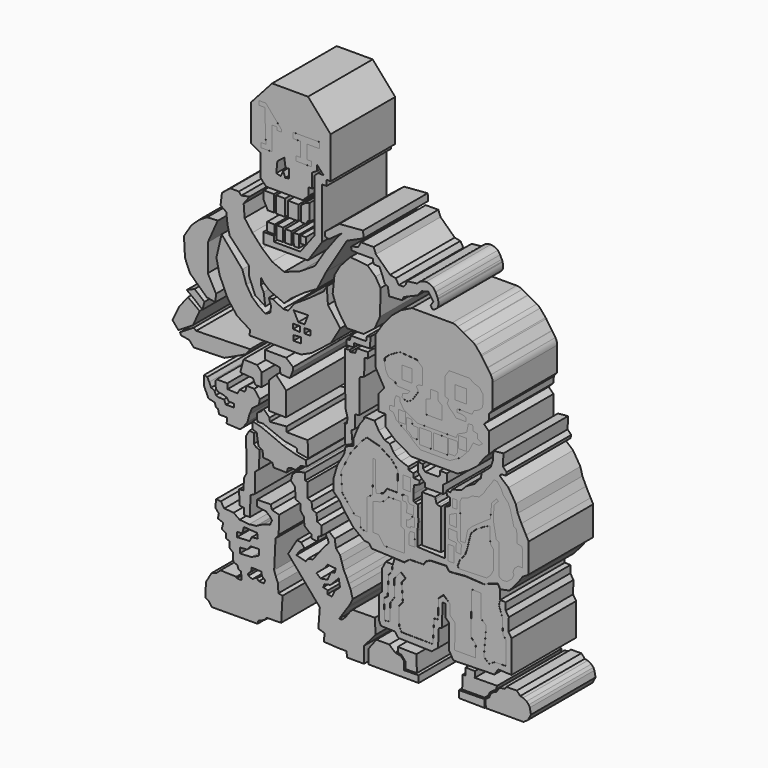
from build123d import *

# Parameters (mm, degrees)
F1_DEPTH       = 12.7
F1_DEPTH_BACK  = 12.7
F0_W           = 2.3451782763
F0_H           = 2.7289353311
F3_DEPTH       = 12.7
F3_DEPTH_BACK  = 12.7
F2_W           = 3.1842617318
F2_H           = 4.0236283094
F2_W_2         = 3.6299433559
F2_H_2         = 4.2267246172
F2_W_3         = 1.8677245826
F2_H_3         = 4.6415366232
F2_W_4         = 1.5032105148
F2_H_4         = 2.5777257979
F2_W_5         = 3.182772547
F2_H_5         = 4.0222080424
F2_W_6         = 3.6285351962
F2_H_6         = 4.2254780419
F2_W_7         = 2.2105854005
F2_H_7         = 3.4294971265
F2_W_8         = 1.8693469465
F2_H_8         = 4.6432167292
F2_W_9         = 1.5042312443
F2_H_9         = 2.5786831975
F2_W_10        = 3.7808120251
F2_H_10        = 4.7481860965
F2_W_11        = 4.3708886951
F2_H_11        = 4.6935402788
F2_W_12        = 2.4654623121
F2_H_12        = 3.6471767817
F2_W_13        = 2.2135460749
F2_H_13        = 3.4322766587
F2_W_14        = 3.7859473377
F2_H_14        = 4.7525740229
F2_W_15        = 4.3766628951
F2_H_15        = 4.6988725662
F2_W_16        = 2.4702642113
F2_H_16        = 3.651695326
F4_T1_DEPTH    = 33.1807281465
F4_T3_DEPTH    = 32.7857254502
F4_T5_DEPTH    = 26.7239636698
F4_T7_DEPTH    = 28.894725654
F4_T9_DEPTH    = 32.1217717721
F4_T11_DEPTH   = 35.0005666731
F4_2_T1_DEPTH  = 25.4
F4_2_T3_DEPTH  = 30.6299842336
F4_2_T5_DEPTH  = 25.6431743127
F4_2_T7_DEPTH  = 26.2196872845
F4_2_T9_DEPTH  = 28.8182396822
F4_2_T11_DEPTH = 30.1563360546


# Not quite as in the source:
# - a fillet or chamfer that OpenCascade refuses, or shapes differently, is made with other operations: its cross-section is extruded or revolved along the edge and cut away or added
# - a feature names something its author has since deleted; it is built from what else it names


with BuildPart() as f1:
    # F0 (on Front) → F1 (new body, two sides)
    with BuildSketch(Plane.XZ) as f1_sk:
        Polygon((-9.5938611776, 66.9106543064), (-16.6862662882, 74.9939456582), (-27.994306758, 74.9939456582), (-34.6385799348, 67.5830319524), (-34.6385799348, 56.2110990286), (-31.6603220999, 54.5591711998), (-31.6603220999, 47.6847961545), (-29.7909770161, 45.815449208), (-18.3336883783, 45.815449208), (-16.5246427059, 47.5641936064), (-16.5246427059, 49.9762557447), (-15.3789138421, 49.9762557447), (-15.3789138421, 54.4385686517), (-13.9103056863, 55.3104877472), (-13.9103056863, 57.1270510554), (-11.8339713663, 54.8590533435), (-13.5205361214, 54.8850011104), (-14.5949935541, 53.9049506187), (-14.5949935541, 37.3129360378), (-17.3938885863, 33.6037576199), (-19.1130582243, 31.3254632056), (-27.4183992296, 31.3254632056), (-27.4183992296, 32.9865328968), (-30.7405348867, 32.9865328968), (-30.7405348867, 29.6643972397), (-16.7492311448, 29.6643972397), (-12.3410113156, 36.1170060933), (-12.3410113156, 52.1527044475), (-10.8716050163, 52.1527044475), (-10.8716050163, 53.877659142), (-9.5938611776, 53.877659142), align=None)
        Polygon((-26.3316370547, 54.0427602828), (-24.165680632, 55.7010732591), (-23.7595625222, 52.9597811401), (-22.728053189, 53.1125976231), (-22.728053189, 50.3538660705), (-23.861091584, 50.2184927464), (-24.5041102171, 51.8768019974), (-25.3163445741, 50.184648484), (-26.6700685024, 50.5569241941), align=None, mode=Mode.SUBTRACT)
        Polygon((-31.4840041101, 57.4934072793), (-29.9422182143, 57.4934072793), (-30.3007718176, 67.6046609879), (-32.0935472846, 67.6046609879), (-32.0935472846, 68.8936337829), (-29.9574602395, 68.8936337829), (-24.9686259777, 63.0946457386), (-24.9686259777, 62.4657310545), (-26.4403745532, 62.4657310545), (-26.5174116939, 63.4554550052), (-28.077730909, 63.4554550052), (-28.077730909, 56.0591891408), (-31.4840041101, 56.0591891408), align=None, mode=Mode.SUBTRACT)
        Polygon((-21.3707555085, 61.8773698807), (-21.3707555085, 63.4141266346), (-21.3707555085, 63.6133402586), (-13.1177809089, 63.6133402586), (-13.1177809089, 61.763536185), (-16.9881414622, 61.763536185), (-16.9881414622, 57.4662983418), (-15.6221324578, 57.4662983418), (-15.6221324578, 55.9295378625), (-20.4316228628, 55.9295378625), (-20.4316228628, 57.4093796313), (-19.0371554345, 57.4093796313), (-19.0371554345, 61.8773698807), align=None, mode=Mode.SUBTRACT)
    extrude(amount=F1_DEPTH)
    extrude(f1_sk.sketch, amount=-F1_DEPTH_BACK)


with BuildPart() as f1b:
    # F0 (on Front) → F1, piece 2 (new body, two sides)
    with BuildSketch(Plane.XZ) as f1_2_sk:
        Polygon((-30.6372623891, 44.5467084646), (-30.6372623891, 44.2908704281), (-30.6372623891, 41.903052479), (-29.358074069, 39.4299551845), (-27.3966528475, 39.4299551845), (-27.3966528475, 44.5467084646), align=None)
    extrude(amount=F1_DEPTH)
    extrude(f1_2_sk.sketch, amount=-F1_DEPTH_BACK)


with BuildPart() as f1c:
    # F0 (on Front) → F1, piece 3 (new body, two sides)
    with BuildSketch(Plane.XZ) as f1_3_sk:
        Polygon((-23.9142030478, 44.4402880967), (-26.7252419144, 44.472232461), (-26.7252419144, 39.3612533808), (-23.9142030478, 39.3612533808), align=None)
    extrude(amount=F1_DEPTH)
    extrude(f1_3_sk.sketch, amount=-F1_DEPTH_BACK)


with BuildPart() as f1d:
    # F0 (on Front) → F1, piece 4 (new body, two sides)
    with BuildSketch(Plane.XZ) as f1_4_sk:
        Polygon((-19.6976456791, 44.1527962685), (-22.9558944702, 44.1847406328), (-22.9558944702, 39.5529158413), (-19.6976456791, 39.5529158413), align=None)
    extrude(amount=F1_DEPTH)
    extrude(f1_4_sk.sketch, amount=-F1_DEPTH_BACK)


with BuildPart() as f1e:
    # F0 (on Front) → F1, piece 5 (new body, two sides)
    with BuildSketch(Plane.XZ) as f1_5_sk:
        Polygon((-17.4935366958, 45.2708229423), (-18.8671126962, 44.2805700004), (-18.8671126962, 39.5529158413), (-17.1741005033, 39.5529158413), (-16.8227199465, 40.5431687832), (-16.1519050598, 40.5431687832), (-16.1519050598, 45.7819215953), align=None)
    extrude(amount=F1_DEPTH)
    extrude(f1_5_sk.sketch, amount=-F1_DEPTH_BACK)


with BuildPart() as f1f:
    # F0 (on Front) → F1, piece 6 (new body, two sides)
    with BuildSketch(Plane.XZ) as f1_6_sk:
        Polygon((-19.0333388746, 33.6037576199), (-17.3938885863, 33.6037576199), (-17.3938885863, 35.8636565506), (-19.0333388746, 35.8636565506), (-19.0333388746, 35.5651788414), align=None)
    extrude(amount=F1_DEPTH)
    extrude(f1_6_sk.sketch, amount=-F1_DEPTH_BACK)


with BuildPart() as f1g:
    # F0 (on Front) → F1, piece 7 (new body, two sides)
    with BuildSketch(Plane.XZ) as f1_7_sk:
        Polygon((-21.2505981326, 35.8636565506), (-21.1653206497, 32.1540087461), (-19.5450149477, 32.1540087461), (-19.5450149477, 35.8636565506), align=None)
    extrude(amount=F1_DEPTH)
    extrude(f1_7_sk.sketch, amount=-F1_DEPTH_BACK)


with BuildPart() as f1h:
    # F0 (on Front) → F1, piece 8 (new body, two sides)
    with BuildSketch(Plane.XZ) as f1_8_sk:
        Polygon((-23.8516163081, 36.0342152417), (-23.8942559808, 32.1966484189), (-21.8475535512, 32.1966484189), (-21.8475535512, 36.0342152417), align=None)
    extrude(amount=F1_DEPTH)
    extrude(f1_8_sk.sketch, amount=-F1_DEPTH_BACK)


with BuildPart() as f1i:
    # F0 (on Front) → F1, piece 9 (new body, two sides)
    with BuildSketch(Plane.XZ) as f1_9_sk:
        Polygon((-26.5379119664, 36.2047739327), (-26.623191312, 32.1966484189), (-24.5338492095, 32.1966484189), (-24.5338492095, 36.2047739327), align=None)
    extrude(amount=F1_DEPTH)
    extrude(f1_9_sk.sketch, amount=-F1_DEPTH_BACK)


with BuildPart() as f1j:
    # F0 (on Front) → F1, piece 10 (new body, two sides)
    with BuildSketch(Plane.XZ) as f1_10_sk:
        with Locations((-28.3500943333, 34.8403062671)):
            Rectangle(F0_W, F0_H)
    extrude(amount=F1_DEPTH)
    extrude(f1_10_sk.sketch, amount=-F1_DEPTH_BACK)


with BuildPart() as f1k:
    # F0 (on Front) → F1, piece 11 (new body, two sides)
    with BuildSketch(Plane.XZ) as f1_11_sk:
        Polygon((-36.9369212724, 38.8479313689), (-35.0333526731, 41.3705967367), (-37.6954227686, 40.775667876), (-38.418225944, 41.6791699827), (-41.128732264, 41.6791699827), (-43.7488853931, 39.6011136472), (-44.2006364465, 35.9871052206), (-42.3936359584, 34.7222052515), (-42.0322343707, 31.4695984125), (-41.3094311953, 28.488041833), (-35.2559685707, 22.1635270864), (-35.2559685707, 19.3626713008), (-33.3586148918, 14.6644618362), (-30.1060080528, 12.5864073634), (-30.6481085718, 16.3811147213), (-31.5516106784, 18.097769469), (-31.42894949, 20.0820728757), (-30.6238532066, 18.9463123679), (-28.6898408085, 17.3346363008), (-24.1771470755, 15.4006257653), (-21.9745226204, 17.4420811236), (-17.7304428071, 20.4505436122), (-13.8624189422, 22.7068904787), (-10.961400345, 28.4014809877), (-4.491341766, 39.0913411975), (0.7715018001, 41.4606525215), (0.5989942583, 43.5738749802), (-6.8465704098, 42.9660752416), (-11.3291051239, 39.3952429295), (-11.3291051239, 38.0276888609), (-10.1135037839, 37.7237871289), (-6.0868188739, 40.610846132), (-7.7582728118, 38.7114658952), (-11.4810559899, 33.6971059442), (-14.5200621337, 28.8346949965), (-19.1545449197, 25.8716642857), (-24.1689067334, 24.0482613444), (-27.9676634818, 25.6437398493), (-31.0826450586, 28.3028688282), (-34.1976247728, 31.6457748413), (-36.6288311779, 34.9127091467), align=None)
    extrude(amount=F1_DEPTH)
    extrude(f1_11_sk.sketch, amount=-F1_DEPTH_BACK)


with BuildPart() as f1l:
    # F0 (on Front) → F1, piece 12 (new body, two sides)
    with BuildSketch(Plane.XZ) as f1_12_sk:
        Polygon((-0.9377481183, 38.5080315173), (-3.0890780035, 37.9343405366), (-3.1607891433, 37.7909205854), (-2.9456561897, 36.9303897023), (-1.2245918624, 36.7869660258), (3.723466536, 36.7869660258), (3.8668890484, 35.3527478874), (5.8030853979, 35.2093242109), (6.663617678, 33.2014150918), (7.3807276785, 31.1935078353), (8.3846813068, 30.6198205799), (8.8149476796, 28.0382242054), (12.8307631239, 28.2533578575), (13.4044513106, 29.3290223926), (15.0538031012, 30.0461333245), (17.7788212895, 31.1935078353), (18.9979076385, 32.7711515129), (21.1492385715, 33.3448387682), (22.7268803865, 31.0500860214), (21.8663476408, 29.8309996724), (22.4400348961, 28.7553351372), (23.6591231078, 29.0421787649), (24.5913658291, 30.7632423937), (24.0176785737, 32.6277278364), (23.0854358524, 34.5639251173), (21.7229258269, 35.7830114663), (18.4959303588, 35.7830114663), (17.6354013383, 34.4205051661), (14.4084058702, 34.0619497001), (13.978138566, 32.9145714641), (13.4044513106, 32.1974642575), (11.8268085644, 32.1257524192), (10.894565843, 33.7033942342), (9.1017913073, 34.0619497001), (4.6557090245, 38.2928960025), (3.938599024, 40.0856733322), (0, 40.0856733322), align=None)
    extrude(amount=F1_DEPTH)
    extrude(f1_12_sk.sketch, amount=-F1_DEPTH_BACK)

    # F4: fillet of radius 3.5186609131 on 6 edges, made by hand

    # F4_s2 → F4_t1 (cut)
    with BuildSketch(Plane.XZ.offset(-16.5903640732)):
        with BuildLine():
            ThreePointArc((24.400289, 30.4104851414), (23.576390538, 29.3978829612), (22.4400348961, 28.7553351372))
            Line((22.4400348961, 28.7553351372), (22.4627084207, 28.6887145614))
            ThreePointArc((22.4627084207, 28.6887145614), (23.065697202, 28.830254444), (23.6752413078, 28.9736762579))
            Line((23.6752413078, 28.9736762579), (23.7210017144, 29.0086611891))
            Line((23.7210017144, 29.0086611891), (24.4621676066, 30.3769675656))
            Line((24.4621676066, 30.3769675656), (24.400289, 30.4104851414))
        make_face()
    extrude(amount=F4_T1_DEPTH, mode=Mode.SUBTRACT)

    # F4_s4 → F4_t3 (cut)
    with BuildSketch(Plane.XZ.offset(-16.3928627251)):
        with BuildLine():
            ThreePointArc((24.1569587579, 32.1750667856), (24.2953412231, 30.792633601), (23.8878265601, 29.4644005581))
            Line((23.8878265601, 29.4644005581), (23.9497051667, 29.4308829823))
            Line((23.9497051667, 29.4308829823), (24.6673152211, 30.7557016546))
            Line((24.6673152211, 30.7557016546), (24.2242200085, 32.1957625344))
            Line((24.2242200085, 32.1957625344), (24.1569587579, 32.1750667856))
        make_face()
    extrude(amount=F4_T3_DEPTH, mode=Mode.SUBTRACT)

    # F4_s6 → F4_t5 (cut)
    with BuildSketch(Plane.XZ.offset(-13.3619818349)):
        with BuildLine():
            ThreePointArc((23.9028073914, 32.8663065517), (24.0084156505, 32.6240965562), (24.0955502986, 32.3746444777))
            Line((24.0955502986, 32.3746444777), (24.1628115492, 32.3953402265))
            Line((24.1628115492, 32.3953402265), (24.0833823898, 32.6534852523))
            Line((24.0833823898, 32.6534852523), (23.9662137839, 32.896835542))
            Line((23.9662137839, 32.896835542), (23.9028073914, 32.8663065517))
        make_face()
    extrude(amount=F4_T5_DEPTH, mode=Mode.SUBTRACT)

    # F4_s8 → F4_t7 (cut)
    with BuildSketch(Plane.XZ.offset(-14.447362827)):
        with BuildLine():
            ThreePointArc((22.5645527671, 35.0299778045), (23.030491922, 34.5226046703), (23.3886490575, 33.9341743347))
            Line((23.3886490575, 33.9341743347), (23.45205545, 33.9647033249))
            Line((23.45205545, 33.9647033249), (23.1427779808, 34.6070491231))
            Line((23.1427779808, 34.6070491231), (22.6114772337, 35.0824228641))
            Line((22.6114772337, 35.0824228641), (22.5645527671, 35.0299778045))
        make_face()
    extrude(amount=F4_T7_DEPTH, mode=Mode.SUBTRACT)

    # F4_s10 → F4_t9 (cut)
    with BuildSketch(Plane.XZ.offset(-16.060885886)):
        with BuildLine():
            ThreePointArc((20.3785714725, 35.7830114663), (21.6343890455, 35.5512787308), (22.724794805, 34.886603534))
            Line((22.724794805, 34.886603534), (22.7717192716, 34.9390485936))
            Line((22.7717192716, 34.9390485936), (21.749812914, 35.8533846845))
            Line((21.749812914, 35.8533846845), (20.3785714725, 35.8533846845))
            Line((20.3785714725, 35.8533846845), (20.3785714725, 35.7830114663))
        make_face()
    extrude(amount=F4_T9_DEPTH, mode=Mode.SUBTRACT)

    # F4_s12 → F4_t11 (cut)
    with BuildSketch(Plane.XZ.offset(-17.5002833365)):
        with BuildLine():
            ThreePointArc((17.6354013383, 34.4205051661), (18.8677869862, 35.4240777234), (20.4160436934, 35.7830114663))
            Line((20.4160436934, 35.7830114663), (20.4160436934, 35.8533846845))
            Line((20.4160436934, 35.8533846845), (18.4959303588, 35.8533846845))
            Line((18.4959303588, 35.8533846845), (18.4364305585, 35.8205902318))
            ThreePointArc((18.4364305585, 35.8205902318), (18.0061660483, 35.1393370817), (17.5797884912, 34.4636282583))
            Line((17.5797884912, 34.4636282583), (17.6354013383, 34.4205051661))
        make_face()
    extrude(amount=F4_T11_DEPTH, mode=Mode.SUBTRACT)


with BuildPart() as f1m:
    # F0 (on Front) → F1, piece 13 (new body, two sides)
    with BuildSketch(Plane.XZ) as f1_13_sk:
        Polygon((2.0290226676, 34.3684926629), (-3.3819169391, 34.9032784963), (-5.0103398971, 33.2014150918), (-6.7701800726, 31.1195589602), (-8.394648321, 28.276739642), (-8.936136961, 22.9972191155), (-7.8531587496, 20.0190264732), (-6.0933185741, 17.1085204929), (-4.4688507915, 14.8748783395), (0.8106696187, 15.0102507323), (4.1949781589, 17.5823252648), (5.9548197314, 21.508121863), (6.0901925899, 29.4274035841), (4.5334086753, 32.0671647787), align=None)
    extrude(amount=F1_DEPTH)
    extrude(f1_13_sk.sketch, amount=-F1_DEPTH_BACK)


with BuildPart() as f1n:
    # F0 (on Front) → F1, piece 14 (new body, two sides)
    with BuildSketch(Plane.XZ) as f1_14_sk:
        Polygon((-37.35839203, 20.4856079072), (-43.8636057079, 28.0750244856), (-45.4980805516, 21.0728552192), (-44.4747321308, 16.553055495), (-41.9163554907, 10.8393486589), (-39.0168614686, 7.087062113), (-34.9234566092, 4.5286854729), (-35.0940153003, 2.908379538), (-18.8909620047, 2.908379538), (-15.6503524631, 4.3581272475), (-9.5305331051, 9.1014830396), (-6.5489741974, 14.1610940918), (-10.4340352118, 19.4014050066), (-10.7954340056, 24.3706665933), (-11.7892883718, 22.6540118456), (-16.6681967676, 19.1303547472), (-20.8243075758, 16.4198484272), (-22.9927096516, 13.7093439698), (-24.5286636055, 13.7093439698), (-27.7812685817, 15.335646458), (-29.0461741388, 15.335646458), (-28.323372826, 13.2575919852), (-28.5944230855, 11.2698879093), (-30.1303770393, 10.5470865965), (-32.2987772524, 11.9926892221), (-34.2864841223, 13.7996925041), (-36.0934883356, 16.6908986866), align=None)
        Polygon((-21.2671738118, 5.9554395266), (-21.2671738118, 7.5206770562), (-18.9672354609, 7.7123385854), (-18.9672354609, 5.9554395266), align=None, mode=Mode.SUBTRACT)
        Polygon((-21.3949494064, 9.1498009861), (-21.3949494064, 10.6511516497), (-19.1588960588, 10.6511516497), (-19.1588960588, 8.9900828898), align=None, mode=Mode.SUBTRACT)
        Polygon((-19.7437535971, 11.6068609059), (-20.9376644343, 13.9094004408), (-21.1935024709, 14.4210755825), (-16.6737027466, 14.506354928), (-17.7823323756, 11.6068609059), align=None, mode=Mode.SUBTRACT)
        Polygon((-17.8172644228, 9.0539706871), (-17.8172644228, 10.5872638524), (-15.9006472677, 10.6511516497), (-15.9006472677, 9.0539706871), align=None, mode=Mode.SUBTRACT)
    extrude(amount=F1_DEPTH)
    extrude(f1_14_sk.sketch, amount=-F1_DEPTH_BACK)


with BuildPart() as f1o:
    # F0 (on Front) → F1, piece 15 (new body, two sides)
    with BuildSketch(Plane.XZ) as f1_15_sk:
        Polygon((-48.2119210064, 24.4022365659), (-45.1531931758, 31.3246250153), (-44.9922047555, 31.4856097102), (-48.4028458595, 31.2973856926), (-50.9676299989, 29.741641134), (-53.3509030938, 27.4967011064), (-55.6977577507, 23.7582940608), (-55.3757883608, 17.8018212318), (-53.8464225829, 14.0991490334), (-50.7876947522, 11.2014058977), (-48.5338903964, 9.1085908934), (-45.7971356809, 8.6256340146), (-45.636150986, 11.0404202715), (-48.2119210064, 15.8699918538), align=None)
    extrude(amount=F1_DEPTH)
    extrude(f1_15_sk.sketch, amount=-F1_DEPTH_BACK)


with BuildPart() as f1p:
    # F0 (on Front) → F1, piece 16 (new body, two sides)
    with BuildSketch(Plane.XZ) as f1_16_sk:
        Polygon((-52.33906582, 10.1660164073), (-54.8434145749, 9.0845925733), (-52.5667332113, 7.4339979328), (-49.8916320503, 5.2142329514), (-49.2655448616, 7.6047494076), align=None)
    extrude(amount=F1_DEPTH)
    extrude(f1_16_sk.sketch, amount=-F1_DEPTH_BACK)


with BuildPart() as f1q:
    # F0 (on Front) → F1, piece 17 (new body, two sides)
    with BuildSketch(Plane.XZ) as f1_17_sk:
        Polygon((-50.790656358, 4.5965607278), (-54.4437915087, 7.2289654054), (-57.129919529, 3.7907224614), (-59.3325421214, -0.6682488602), (-57.4522539973, -2.8708733153), (-52.8321154416, 0), align=None)
    extrude(amount=F1_DEPTH)
    extrude(f1_17_sk.sketch, amount=-F1_DEPTH_BACK)


with BuildPart() as f1r:
    # F0 (on Front) → F1, piece 18 (new body, two sides)
    with BuildSketch(Plane.XZ) as f1_18_sk:
        Polygon((-52.617225796, -0.6145262741), (-56.9150298834, -3.3006537706), (-56.6464141011, -4.0527693927), (-54.0677346289, -4.4825496152), (-52.617225796, -6.094226148), (-43.0546104908, -5.8793355711), (-39.5626462996, -4.267659504), (-36.2318493426, -2.655983204), (-34.8887853324, -0.8294165018), (-51.8651083112, -1.2591967825), align=None)
    extrude(amount=F1_DEPTH)
    extrude(f1_18_sk.sketch, amount=-F1_DEPTH_BACK)


with BuildPart() as f1s:
    # F0 (on Front) → F1, piece 19 (new body, two sides)
    with BuildSketch(Plane.XZ) as f1_19_sk:
        Polygon((-23.6031040549, 0.4885619273), (-30.1950573921, 0.5392691819), (-30.1950573921, -2.1482193843), (-25.5299843848, -2.8074146248), (-25.3778602928, -4.5821708627), (-22.4875435233, -4.7850008123), (-21.524105221, -2.7567071375), (-21.3719829917, -1.3876094017), align=None)
    extrude(amount=F1_DEPTH)
    extrude(f1_19_sk.sketch, amount=-F1_DEPTH_BACK)


with BuildPart() as f1t:
    # F0 (on Front) → F1, piece 20 (new body, two sides)
    with BuildSketch(Plane.XZ) as f1_20_sk:
        Polygon((-36.8002168834, -4.3107029051), (-36.9612015784, -4.3107029051), (-38.0076095462, -8.2548540086), (-33.9829660952, -8.5768252611), (-33.2585312426, -10.1866824552), (-31.3267037272, -10.1866824552), (-31.2462095171, -6.0815461911), (-32.695081085, -4.4716885313), align=None)
    extrude(amount=F1_DEPTH)
    extrude(f1_20_sk.sketch, amount=-F1_DEPTH_BACK)


with BuildPart() as f1u:
    # F0 (on Front) → F1, piece 21 (new body, two sides)
    with BuildSketch(Plane.XZ) as f1_21_sk:
        Polygon((-28.9138779044, -7.434383966), (-29.0096011013, -7.434383966), (-29.0096011013, -15.9537047148), (-23.6491281539, -16.049426049), (-23.5534086823, -8.5830567405), (-26.7122555524, -5.2327625453), align=None)
    extrude(amount=F1_DEPTH)
    extrude(f1_21_sk.sketch, amount=-F1_DEPTH_BACK)


with BuildPart() as f1v:
    # F0 (on Front) → F1, piece 22 (new body, two sides)
    with BuildSketch(Plane.XZ) as f1_22_sk:
        Polygon((-5.1528443582, -11.6437776014), (-4.9752146006, -17.6448337734), (-2.6907407378, -16.5448998462), (-3.0455661472, -12.9111642018), (-1.8998369342, -12.1272439137), (-1.929987804, -8.1473439932), (-0.5732035497, -7.9362886027), (-0.42929349, 2.6036400814), (0.9762255359, 3.2425122336), (0.9992049308, 8.3681419492), (2.2052354179, 8.7299505249), (2.0846324041, 10.4183927178), (-1.2922529131, 10.3580914438), (-1.8349663587, 8.9108552784), (-3.40280612, 8.6394986138), (-3.5535597708, 9.21236258), (-5.0912485458, 8.9711565524), (-4.961182829, -7.0438971743), (-4.7858525068, -7.9941847362), (-4.2383526452, -9.9451867864), (-4.5139719732, -11.4521170035), align=None)
    extrude(amount=F1_DEPTH)
    extrude(f1_22_sk.sketch, amount=-F1_DEPTH_BACK)


with BuildPart() as f1w:
    # F0 (on Front) → F1, piece 23 (new body, two sides)
    with BuildSketch(Plane.XZ) as f1_23_sk:
        Polygon((-3.4961928613, 11.9555769488), (-4.6345340088, 11.6994502023), (-4.6345340088, 10.1626897231), (-2.32939329, 10.2765234187), (-2.2155591287, 11.4717818797), (2.7931416407, 11.6140749305), (2.9354346916, 14.9437226355), (1.7970931949, 14.6591365337), (1.5694251051, 13.2362106815), (-3.2685245387, 13.2362106815), align=None)
    extrude(amount=F1_DEPTH)
    extrude(f1_23_sk.sketch, amount=-F1_DEPTH_BACK)


with BuildPart() as f1x:
    # F0 (on Front) → F1, piece 24 (new body, two sides)
    with BuildSketch(Plane.XZ) as f1_24_sk:
        Polygon((-32.6734371483, -17.6987983286), (-32.6734371483, -19.6284465492), (-32.5862728059, -20.1711598784), (-30.7437889278, -20.1108586043), (-28.5126324743, -21.0153814405), (-24.2312233895, -22.7038245648), (-20.2513244003, -23.4274435788), (-20.1307218522, -24.5128702372), (-16.6332330555, -25.1158848405), (-16.8141368777, -20.1108586043), (-23.4473049641, -20.0505573303), (-23.4473049641, -18.4827186167), (-28.6935362965, -18.9048293978), (-28.8141407073, -17.8194008768), (-30.6231863797, -16.0103552043), (-31.3468053937, -16.8545767665), align=None)
    extrude(amount=F1_DEPTH)
    extrude(f1_24_sk.sketch, amount=-F1_DEPTH_BACK)


with BuildPart() as f1y:
    # F0 (on Front) → F1, piece 25 (new body, two sides)
    with BuildSketch(Plane.XZ) as f1_25_sk:
        Polygon((-31.2966257334, -21.257204935), (-34.0757220984, -20.5111056566), (-34.0757220984, -22.7471590042), (-32.8299216926, -23.1943689287), (-32.2868786752, -26.7720539123), (-30.9771914035, -27.6025887579), (-30.7855289429, -29.5192059129), (-28.9008561522, -29.6469796449), (-27.8467163444, -29.9983602017), (-27.5272801518, -31.1802737415), (-23.4384965152, -31.2441606075), (-23.023230955, -29.9025289714), (-21.7774286866, -29.4872615486), (-20.5955151469, -29.5830927789), (-19.7330377996, -28.6886710674), (-18.9983341843, -27.9220249504), (-17.1775482595, -27.6025887579), (-17.3692107201, -25.8776322007), (-20.946893841, -25.1543261111), (-24.3968050927, -24.1640750319), (-27.3995064199, -22.8863302618), align=None)
    extrude(amount=F1_DEPTH)
    extrude(f1_25_sk.sketch, amount=-F1_DEPTH_BACK)


with BuildPart() as f1z:
    # F0 (on Front) → F1, piece 26 (new body, two sides)
    with BuildSketch(Plane.XZ) as f1_26_sk:
        Polygon((-43.0968850851, -17.3945352435), (-44.8567271233, -17.3945352435), (-45.6112548709, -17.0357543975), (-46.1307689548, -15.951551497), (-47.1697971225, -15.4546266422), (-47.7570705116, -14.0993734822), (-48.344347626, -12.8796454519), (-49.3616610765, -12.6537699252), (-49.3616610765, -15.761744231), (-47.9702912271, -18.7482573092), (-45.9973849356, -19.1603135318), (-45.6689596176, -20.3727260232), (-44.9827052653, -20.6235628575), (-44.6536689997, -22.0648795366), (-42.1492792666, -22.0648795366), (-42.2846525908, -23.8247197121), (-38.0881093442, -24.0277796984), (-37.2081883252, -23.2832320035), (-35.7190929353, -21.2526451796), (-35.1099185646, -18.9513172954), (-34.2976860702, -16.9884171337), (-32.1317277849, -15.2962636203), (-31.8609811366, -13.6717958376), (-33.6208231747, -11.3704660907), (-35.9221510589, -11.3027794287), (-36.531329155, -13.1303062662), (-38.155797869, -13.0626205355), (-38.9003455639, -14.3486568704), (-42.0139059424, -14.2132854089), (-42.0815944672, -12.5888166949), (-45.3982166946, -12.5888166949), (-45.7513257861, -13.1409596652), (-45.6944070756, -15.1330558583), (-44.9921004474, -15.9054398537), (-43.3676317334, -16.1761846393), (-42.2846525908, -16.5823008865), (-41.6077896953, -17.4622200429), (-39.9833209813, -17.529906705), (-39.9156361818, -18.6128858477), (-42.5553955138, -18.6805725098), align=None)
    extrude(amount=F1_DEPTH)
    extrude(f1_26_sk.sketch, amount=-F1_DEPTH_BACK)


with BuildPart() as f1ba:
    # F0 (on Front) → F1, piece 27 (new body, two sides)
    with BuildSketch(Plane.XZ) as f1_27_sk:
        Polygon((-33.6043462157, -23.650649935), (-35.135909915, -23.435274139), (-36.1285246909, -25.1578874886), (-36.0905379057, -35.6804467738), (-36.8502885103, -37.1619611979), (-36.9642525911, -40.580842644), (-38.3318029344, -40.6948067248), (-38.2938161492, -45.1773405075), (-36.8882752955, -45.3292913735), (-36.8123017251, -47.3046451807), (-34.9509119987, -47.3426319659), (-34.7989611328, -41.1886461079), (-33.4396325052, -40.4247939587), (-33.4396325052, -34.3261547387), (-32.0843793452, -33.1516042352), (-31.9770611823, -27.7427956462), (-33.0539382994, -27.3120421916), (-33.7239988148, -26.6180541366), align=None)
    extrude(amount=F1_DEPTH)
    extrude(f1_27_sk.sketch, amount=-F1_DEPTH_BACK)


with BuildPart() as f1bb:
    # F0 (on Front) → F1, piece 28 (new body, two sides)
    with BuildSketch(Plane.XZ) as f1_28_sk:
        Polygon((-18.8277959824, -29.6179540455), (-20.5805432051, -30.192617327), (-21.6056704521, -31.1802737415), (-22.0880825073, -33.0267883837), (-20.76144889, -34.3534238636), (-20.6408444792, -37.7303063869), (-19.0127044916, -38.3936241269), (-19.0730057657, -40.3232723475), (-17.9272778332, -41.8308116496), (-17.860205844, -44.0748855472), (-16.3803622127, -45.3839786351), (-15.6404413283, -45.7823984325), (-15.5835244805, -46.9207391143), (-13.6483442038, -47.1484065056), (-13.5345105082, -45.7823984325), (-12.3961688951, -45.1563112438), (-12.510003522, -42.3673763871), (-13.8760125265, -41.6843704879), (-13.9898471534, -39.4076891243), (-15.29893931, -38.9523506165), (-15.5835244805, -36.7895029485), (-16.8357007205, -36.2203344703), (-16.8357007205, -31.7238867283), (-17.5756216049, -31.5531343222), (-17.6325384527, -29.3902866542), align=None)
    extrude(amount=F1_DEPTH)
    extrude(f1_28_sk.sketch, amount=-F1_DEPTH_BACK)


with BuildPart() as f1bc:
    # F0 (on Front) → F1, piece 29 (new body, two sides)
    with BuildSketch(Plane.XZ) as f1_29_sk:
        Polygon((-28.4168235958, -41.6801795363), (-32.7146276832, -41.7402908206), (-32.7146276832, -43.6743050814), (-29.9210548401, -44.0503619611), (-28.631715104, -45.1248139143), (-28.040766716, -45.9843724966), (-28.631715104, -47.3811589181), (-30.6731704623, -47.9183867574), (-32.9832397401, -49.100279808), (-35.1858660579, -49.3688955903), (-38.1943285465, -49.100279808), (-40.0746166706, -47.7572157979), (-43.0293567479, -47.5423261523), (-44.103808701, -45.9306500852), (-45.6080399454, -45.8232052624), (-45.8229295909, -48.2407212257), (-44.7484776378, -49.5300628245), (-45.0170896947, -50.9805716574), (-43.3516912162, -51.6252405941), (-43.7814742327, -53.4518063068), (-42.4921326339, -54.2039237916), (-42.4921326339, -55.6007102132), (-41.4176806808, -56.0842119157), (-41.3639582694, -57.9107776284), (-40.3432287276, -58.770339936), (-40.1820614934, -61.2953007221), (-38.8927198946, -61.9399696589), (-38.5166630149, -63.0144178867), (-37.7645455301, -63.2293075323), (-37.5496558845, -65.6468272209), (-39.0538871288, -65.5931010842), (-39.215054363, -65.2170479298), (-44.2112535238, -65.0558769703), (-45.5005951226, -66.237770021), (-47.0048263669, -66.7212754488), (-48.7776696682, -69.7233527899), (-48.9925593138, -74.1285979748), (-47.9181073606, -74.7732669115), (-46.8973815441, -76.1163309216), (-32.553460449, -76.0626122355), (-32.284848392, -75.0418826938), (-31.3178412616, -74.7195482254), (-30.2433911711, -74.2360427976), (-29.8136100173, -73.483929038), (-25.1397490501, -73.3764842153), (-24.7099678963, -65.7478794456), (-25.9993094951, -65.4792711139), (-26.1604785919, -62.7394169569), (-26.85886994, -60.9665736556), (-27.3423735052, -59.5160648227), (-26.9125942141, -50.5981221795), (-25.9455870837, -49.3087805808), (-25.7306974381, -43.6679162085), (-28.040766716, -43.0769659579), align=None)
        Polygon((-34.1644622386, -64.2259716988), (-35.4741513729, -63.714876771), (-35.5060957372, -63.0760043859), (-34.579731524, -62.2454695404), (-34.451957792, -61.0954985023), (-31.3534252346, -61.2232722342), (-31.1937071383, -62.3732432723), (-30.1395691931, -63.3315518498), (-30.5548347533, -64.2259716988), (-32.1839600801, -64.1620829701), (-32.7589437366, -63.5870993137), (-33.2380980253, -63.5870993137), align=None, mode=Mode.SUBTRACT)
        Polygon((-38.1465218961, -58.3931319416), (-38.1465218961, -56.7442439497), (-35.8651801944, -56.5861277282), (-34.8487384617, -55.3438141942), (-32.1156457067, -55.2308782935), (-32.0478826761, -57.0378787816), (-34.487336874, -58.2124330103), align=None, mode=Mode.SUBTRACT)
        Polygon((-39.0662886202, -54.2039237916), (-39.0662886202, -52.7116432786), (-37.3587757349, -52.5978058577), (-36.8465222418, -50.6626293063), (-32.6915755868, -50.9472116828), (-32.4639081955, -52.483972162), (-34.3990884721, -52.7116432786), (-35.0251756608, -53.963817656), align=None, mode=Mode.SUBTRACT)
    extrude(amount=F1_DEPTH)
    extrude(f1_29_sk.sketch, amount=-F1_DEPTH_BACK)


with BuildPart() as f1bd:
    # F0 (on Front) → F1, piece 30 (new body, two sides)
    with BuildSketch(Plane.XZ) as f1_30_sk:
        Polygon((-19.426131621, -51.6865924001), (-17.7577332582, -50.3934485057), (-18.8531130552, -49.0724369884), (-20.1647710055, -48.8816089928), (-22.9407288134, -53.5720214248), (-12.9855694249, -65.1544630527), (-13.4641826153, -71.1849927902), (-11.5497289225, -71.7593356967), (-11.6454521194, -74.2481201887), (-6.9550401531, -74.5352879167), (-4.6576941386, -74.5352879167), (-4.3705268763, -76.2583017349), (0.8942213608, -76.2583017349), (0.8942206623, -71.2807178497), (4.5316843316, -67.0689195395), (4.3402379379, -62.3785071075), (-2.7432409115, -62.474232167), (-3.6047447938, -63.4314566851), (-4.8491400667, -65.1544705033), (-5.9978123754, -66.3031414151), (-6.8593169563, -66.3031414151), (-5.9183971025, -64.8603662848), (-4.3988940306, -62.581114471), (-3.7004679907, -61.6127252579), (-2.6475179475, -59.5068261027), (-3.3175775316, -57.0180378854), (-3.8919141516, -55.6779205799), (-4.4662486762, -54.3378032744), (-5.4234764539, -52.4233467877), (-6.0935355723, -50.3174476326), (-6.6678719595, -48.5944412649), (-7.9122660682, -47.1585988998), (-8.2951579243, -44.6698106825), (-10.0181661546, -43.2339683175), (-11.1668379977, -44.2869178951), (-10.4010561481, -45.6270352006), (-10.2167800069, -46.425241977), (-12.3155107722, -48.8816089928), (-15.1871917769, -52.6147931814), (-16.7187545449, -52.9019609094), (-17.3888131976, -53.8591891527), (-20.3562173992, -53.0934073031), align=None)
        Polygon((-10.4784592986, -59.6494115889), (-11.9485352188, -59.2550002038), (-11.518268846, -58.2510456443), (-9.6537834033, -57.8566379845), (-7.0363315754, -55.1674738526), (-6.6419215873, -57.6056502759), (-8.2195624709, -58.9681565762), (-9.1876611114, -60.9402097762), (-10.5860261247, -60.7250779867), align=None, mode=Mode.SUBTRACT)
        Polygon((-12.714728713, -57.0676513016), (-14.0428608283, -55.9809990227), (-13.1171932444, -55.1760718226), (-11.547582224, -53.8881830871), (-10.5414213613, -52.5198057294), (-7.9656485468, -52.7612827718), (-8.3278669044, -54.0894158185), (-9.4950133935, -54.2906485498), (-10.5414213613, -56.7054338753), align=None, mode=Mode.SUBTRACT)
    extrude(amount=F1_DEPTH)
    extrude(f1_30_sk.sketch, amount=-F1_DEPTH_BACK)


with BuildPart() as f1be:
    # F0 (on Front) → F1, piece 31 (new body, two sides)
    with BuildSketch(Plane.XZ) as f1_31_sk:
        Polygon((-29.9574602395, 68.8925981522), (-32.0922508836, 68.8925981522), (-32.0922508836, 67.6055178046), (-30.2996076643, 67.6055178046), (-29.939731583, 57.4920475483), (-31.483117491, 57.4920475483), (-31.483117491, 56.0601837933), (-28.0790179968, 56.0601837933), (-28.0956011266, 63.473932445), (-26.5090446919, 63.4602755308), (-26.436150074, 62.4692924321), (-24.9725058675, 62.4692924321), (-24.9725058675, 63.093483448), align=None)
    extrude(amount=F1_DEPTH)
    extrude(f1_31_sk.sketch, amount=-F1_DEPTH_BACK)


with BuildPart() as f1bf:
    # F0 (on Front) → F1, piece 32 (new body, two sides)
    with BuildSketch(Plane.XZ) as f1_32_sk:
        Polygon((-13.1213907152, 63.6110603809), (-21.3671550155, 63.6095330119), (-21.3671550155, 61.8804320693), (-19.0351754427, 61.8804320693), (-19.0351754427, 57.4064180255), (-20.4279664904, 57.4064180255), (-20.4279664904, 55.9322498739), (-15.6266130507, 55.9322498739), (-15.6266130507, 57.4618503451), (-16.9916376472, 57.4618503451), (-16.9916376472, 61.7666766047), (-13.1213907152, 61.7666766047), align=None)
    extrude(amount=F1_DEPTH)
    extrude(f1_32_sk.sketch, amount=-F1_DEPTH_BACK)


with BuildPart() as f3:
    # F2 (on Front) → F3 (new body, two sides)
    with BuildSketch(Plane.XZ) as f3_sk:
        Polygon((19.411213696, -14.8924924433), (17.8433749825, -14.8924924433), (17.8433749825, -17.7266635001), (18.9891029149, -19.0532971174), (20.0142282993, -19.8975186795), (20.0142282993, -21.2241522968), (25.8031748235, -21.2241522968), (25.8031748235, -18.5708850622), (26.948902756, -17.7266635001), (26.948902756, -15.0733962655), (24.7780475765, -15.0733962655), (24.7780475765, -16.4000298828), (24.1750329733, -16.8824419379), (20.1951339841, -16.8824419379), (19.411213696, -16.1588247865), align=None)
    extrude(amount=F3_DEPTH)
    extrude(f3_sk.sketch, amount=-F3_DEPTH_BACK)


with BuildPart() as f3b:
    # F2 (on Front) → F3, piece 2 (new body, two sides)
    with BuildSketch(Plane.XZ) as f3_2_sk:
        Polygon((23.2366155833, -22.8002108634), (19.1131997854, -22.8002108634), (19.1131997854, -37.5137813389), (25.1433514059, -37.5137813389), (25.1433514059, -24.9107647687), (24.2991298437, -24.8504634947), (23.6961152405, -24.5489552617), (23.3946070075, -23.2826229185), align=None)
    extrude(amount=F3_DEPTH)
    extrude(f3_2_sk.sketch, amount=-F3_DEPTH_BACK)


with BuildPart() as f3c:
    # F2 (on Front) → F3, piece 3 (new body, two sides)
    with BuildSketch(Plane.XZ) as f3_3_sk:
        Polygon((9.8529430106, -45.790258795), (7.7470429242, -45.790258795), (6.6309138201, -47.9049906135), (6.5706125461, -54.4175542891), (5.5454866961, -55.5029809475), (5.6057879701, -62.5582560897), (6.2045394443, -64.0260279179), (10.657816194, -64.1292333603), (11.696241796, -65.5733346939), (22.1887063235, -65.8748447895), (24.1786558181, -64.3070042133), (24.419862777, -58.6386583745), (25.3846868873, -58.3371520042), (25.6258919835, -51.2215718627), (26.6044139862, -51.2464530766), (26.5086907893, -55.0753623247), (27.6573635638, -56.2240332365), (27.6573635638, -63.8818517327), (28.9974808693, -66.1791935563), (41.9200435281, -65.8920258284), (43.0687181652, -64.0732944012), (47.2805164754, -64.2647370696), (47.2805164754, -54.1181340814), (46.3232882321, -52.5865703821), (46.4190095663, -48.5662184656), (45.4617850482, -47.0346547663), (45.4617850482, -44.7373092175), (43.7387749553, -44.6415878832), (43.3558858931, -46.2688729167), (44.4088354707, -49.2362752557), (44.6002818644, -54.0224127471), (45.5575101078, -55.0753623247), (45.5575101078, -62.3502843082), (42.0157685876, -62.4460093677), (40.1970371604, -63.4989589453), (38.5697484016, -62.0631165802), (39.3355339766, -53.160905838), (37.6125238836, -51.7250671983), (37.6125238836, -44.7373092175), (34.7408428788, -44.6415878832), (34.5494002104, -57.9470433295), (36.0809601843, -59.3828819692), (35.8895137906, -63.2117912173), (29.3803717941, -63.2117912173), (29.5718181878, -55.6496977806), (27.9445312917, -54.0224127471), (27.9445312917, -50.8635602891), (25.9343553334, -49.1405539215), (24.4027916342, -50.480671227), (24.2113471031, -56.4154796302), (22.9669511318, -56.6069222987), (22.584060207, -63.7861266732), (12.7246240154, -63.6904016137), (11.9588421658, -62.254562974), (11.8631189689, -56.7026473582), (13.1075140089, -55.1710836589), (12.7246240154, -49.8106107116), (13.969018124, -48.3747720718), (12.4374544248, -47.1303761005), (10.4272784665, -49.6191680431), (10.5230016634, -54.7881908715), (9.1828834265, -56.7026473582), (9.087161161, -61.967395246), (7.364152465, -62.1588379145), (7.1727074683, -56.0325868428), (8.3298254758, -55.1587231457), (8.6085479707, -49.1405539215), (9.6614966169, -47.8004366159), align=None)
    extrude(amount=F3_DEPTH)
    extrude(f3_3_sk.sketch, amount=-F3_DEPTH_BACK)


with BuildPart() as f3d:
    # F2 (on Front) → F3, piece 4 (new body, two sides)
    with BuildSketch(Plane.XZ) as f3_4_sk:
        Polygon((2.2517784964, -71.7037245631), (2.2517784964, -75.5369588733), (2.2456638981, -75.9565010667), (18.095811829, -75.9841650724), (18.031924963, -73.8758891821), (13.4540820119, -73.9403673525), (13.5598191991, -71.5120583773), (12.5376228243, -70.3620910645), (10.6848934665, -69.9787661433), (8.8321631774, -68.3176964521), (4.8072678037, -68.3176964521), align=None)
    extrude(amount=F3_DEPTH)
    extrude(f3_4_sk.sketch, amount=-F3_DEPTH_BACK)


with BuildPart() as f3e:
    # F2 (on Front) → F3, piece 5 (new body, two sides)
    with BuildSketch(Plane.XZ) as f3_5_sk:
        Polygon((11.509006843, -68.1123957038), (11.53915748, -68.3536008), (11.53915748, -69.68023628), (12.6245850697, -69.8912888765), (13.8909174129, -71.3083744049), (13.92106805, -73.4792277217), (17.5391584635, -73.4189301729), (17.3884052783, -68.2329982519), align=None)
    extrude(amount=F3_DEPTH)
    extrude(f3_5_sk.sketch, amount=-F3_DEPTH_BACK)


with BuildPart() as f3f:
    # F2 (on Front) → F3, piece 6 (new body, two sides)
    with BuildSketch(Plane.XZ) as f3_6_sk:
        Polygon((38.7321710587, -73.72418046), (30.7547785342, -73.8381445408), (30.7547785342, -76.0414227843), (38.808144629, -76.1553868651), align=None)
    extrude(amount=F3_DEPTH)
    extrude(f3_6_sk.sketch, amount=-F3_DEPTH_BACK)


with BuildPart() as f3g:
    # F2 (on Front) → F3, piece 7 (new body, two sides)
    with BuildSketch(Plane.XZ) as f3_7_sk:
        Polygon((35.7636064291, -66.9536069036), (32.8658632934, -66.8731182814), (32.8658632934, -69.1269189119), (31.8596996367, -69.2074075341), (31.7792072892, -73.3125433326), (38.8223342597, -73.2723027468), (39.8687422276, -72.427123785), (40.4724404216, -71.3002234697), (41.1968752742, -70.6965252757), (42.3237755895, -69.9720904231), (42.7664853632, -68.7244534492), (35.7233583927, -68.8049420714), align=None)
    extrude(amount=F3_DEPTH)
    extrude(f3_7_sk.sketch, amount=-F3_DEPTH_BACK)


with BuildPart() as f3h:
    # F2 (on Front) → F3, piece 8 (new body, two sides)
    with BuildSketch(Plane.XZ) as f3_8_sk:
        Polygon((40.251083672, -72.7893412113), (39.3052920699, -73.4936520457), (39.1395650804, -73.6936181784), (39.2027460039, -76.079569757), (51.0757006705, -76.0237947106), (52.4053946137, -75.092881918), (53.3972711746, -73.2598043978), (53.0112311244, -71.4450851083), (52.6883378625, -70.7233175635), (52.0235523582, -70.0205489993), (50.9029217064, -69.4317370653), (50.0102117658, -69.2038163543), (48.9275641739, -68.0451914668), (45.6606335938, -68.0831819773), (45.201394707, -68.7848255038), (43.5311682522, -69.0061748028), (42.5652526319, -70.4550519586), (41.6597090662, -70.8172693849), (40.7944098115, -71.5618282557), align=None)
    extrude(amount=F3_DEPTH)
    extrude(f3_8_sk.sketch, amount=-F3_DEPTH_BACK)


with BuildPart() as f3i:
    # F2 (on Front) → F3, piece 9 (new body, two sides)
    with BuildSketch(Plane.XZ) as f3_9_sk:
        Polygon((4.8100892454, -27.8926938772), (4.8788301647, -27.7793295681), (6.9559456266, -27.0710128224), (8.171393536, -25.3861583769), (11.4074870944, -25.4249107093), (11.5326540545, -19.3315073848), (9.6515780315, -16.9598422945), (5.6938042647, -14.4064399843), (1.7834793543, -13.359323144), (0.0197774447, -15.0459936151), (-3.1720004044, -19.0298762172), (-6.3057861459, -25.3135934472), (-5.9224626218, -31.1912186444), (-1.980755711, -36.0438488424), (-0.18749437, -36.0453985631), (-0.104695045, -39.1537784858), (1.8284186246, -39.4873106011), (1.8458900095, -39.4903250477), (1.8498733407, -29.7824908048), (3.6118254066, -28.6000333726), (3.7727496209, -18.4618160129), (3.7727496209, -18.448041752), (4.5599858277, -18.4956751764), (4.4624623843, -25.9686578065), align=None)
    extrude(amount=F3_DEPTH)
    extrude(f3_9_sk.sketch, amount=-F3_DEPTH_BACK)


with BuildPart() as f3j:
    # F2 (on Front) → F3, piece 10 (new body, two sides)
    with BuildSketch(Plane.XZ) as f3_10_sk:
        Polygon((12.5512035929, -27.5318897338), (8.7034376338, -27.6120528579), (7.410542873, -29.0550756119), (6.0419713729, -29.779612506), (3.7883551914, -30.3430166095), (3.7883551914, -38.9545334723), (5.4785431724, -39.0350180932), (7.2494158521, -41.53034091), (13.6876897886, -41.53034091), (13.6782713234, -35.0915119052), (12.4707330288, -34.2913835954), align=None)
    extrude(amount=F3_DEPTH)
    extrude(f3_10_sk.sketch, amount=-F3_DEPTH_BACK)


with BuildPart() as f3k:
    # F2 (on Front) → F3, piece 11 (new body, two sides)
    with BuildSketch(Plane.XZ) as f3_11_sk:
        Polygon((8.8738944357, 11.8528466412), (7.4505838566, 10.5184940621), (7.4110946494, 9.1180661693), (7.7724962372, 7.1755368263), (8.5851195088, 5.6405814991), (10.6631761153, 4.962954689), (11.2955628349, 4.0595442914), (15.4081759974, 3.8787701633), (14.6419124615, 2.9719617509), (13.0144953728, 2.4746954441), (12.8904338714, 1.4012731254), (14.2766190693, 0.730538289), (15.9806408657, 1.5377065266), (18.0044658619, 4.5734448358), (17.709183215, 5.3677497596), (17.2794390956, 5.8452422959), (18.0364142214, 6.5265212356), (19.2315187305, 6.7085986957), (19.2264536499, 11.7355822865), (17.5550207706, 13.286102042), (12.1082141995, 13.6946121137), align=None)
        with Locations((14.4296702929, 8.3201155066)):
            Rectangle(F2_W, F2_H, mode=Mode.SUBTRACT)
    extrude(amount=F3_DEPTH)
    extrude(f3_11_sk.sketch, amount=-F3_DEPTH_BACK)


with BuildPart() as f3l:
    # F2 (on Front) → F3, piece 12 (new body, two sides)
    with BuildSketch(Plane.XZ) as f3_12_sk:
        Polygon((26.3629853725, 11.6480914876), (26.365365833, 6.0368538834), (27.5196485555, 5.6154328279), (27.0641141025, 4.3627084233), (27.8609518347, 3.2243675087), (28.8273151964, 2.3148490643), (29.9091748893, 1.1760494672), (33.0383120829, 1.1760494672), (33.0383120829, 2.3133222744), (31.843919307, 2.7683301984), (30.1350746304, 2.8822531458), (30.1350746304, 3.8516142422), (34.9162829847, 3.8516142422), (35.4280397296, 5.0457133912), (37.0792179113, 5.7291732426), (38.2171032441, 6.8670590408), (38.3309369397, 10.5097498745), (37.1933562092, 12.0454853497), (35.3158600628, 12.6713173985), (34.1199375689, 13.5824959091), (27.6894114359, 13.5824959091), align=None)
        with Locations((31.2793934718, 8.2185673527)):
            Rectangle(F2_W_2, F2_H_2, mode=Mode.SUBTRACT)
    extrude(amount=F3_DEPTH)
    extrude(f3_12_sk.sketch, amount=-F3_DEPTH_BACK)


with BuildPart() as f3m:
    # F2 (on Front) → F3, piece 13 (new body, two sides)
    with BuildSketch(Plane.XZ) as f3_13_sk:
        Polygon((13.1141859401, -19.9630289751), (13.1142763421, -23.8833520561), (15.5840891304, -23.9370453584), (15.5840891304, -20.0167223811), align=None)
    extrude(amount=F3_DEPTH)
    extrude(f3_13_sk.sketch, amount=-F3_DEPTH_BACK)


with BuildPart() as f3n:
    # F2 (on Front) → F3, piece 14 (new body, two sides)
    with BuildSketch(Plane.XZ) as f3_14_sk:
        Polygon((14.6602072638, -25.3948126497), (12.9216276109, -25.4025906324), (12.9615227783, -26.0908916892), (12.9615227783, -27.1095056087), (14.028663747, -27.1934978664), (14.4094737044, -27.6758577675), (14.3080983809, -30.1088692563), (16.4102148265, -30.1088692563), (16.5622463779, -27.4229816162), (15.3675985136, -27.3553599609), (14.8375943041, -26.9659552723), align=None)
    extrude(amount=F3_DEPTH)
    extrude(f3_14_sk.sketch, amount=-F3_DEPTH_BACK)


with BuildPart() as f3o:
    # F2 (on Front) → F3, piece 15 (new body, two sides)
    with BuildSketch(Plane.XZ) as f3_15_sk:
        Polygon((16.7892678302, -33.40784089), (16.7178865522, -30.6571312249), (16.0966416589, -30.5854492649), (15.5697613955, -31.3995219767), (14.8279098794, -31.9738574326), (14.3259083852, -31.9733321667), (14.3259083852, -33.934533596), (15.4256401584, -33.934533596), (15.6650380421, -33.3839205131), align=None)
    extrude(amount=F3_DEPTH)
    extrude(f3_15_sk.sketch, amount=-F3_DEPTH_BACK)


with BuildPart() as f3p:
    # F2 (on Front) → F3, piece 16 (new body, two sides)
    with BuildSketch(Plane.XZ) as f3_16_sk:
        Polygon((16.8296981012, -34.8238106071), (15.4489697888, -34.8470285535), (15.1187284069, -35.6099568307), (15.1187284069, -38.7751497328), (16.8961550268, -38.7450258294), align=None)
    extrude(amount=F3_DEPTH)
    extrude(f3_16_sk.sketch, amount=-F3_DEPTH_BACK)


with BuildPart() as f3q:
    # F2 (on Front) → F3, piece 17 (new body, two sides)
    with BuildSketch(Plane.XZ) as f3_17_sk:
        Polygon((31.2190782279, -32.4576869607), (32.7085070312, -32.4576869607), (33.4891026329, -28.6585802484), (34.8305478692, -27.2532589734), (36.5037880838, -26.0431521094), (38.9426494261, -24.3269164189), (40.6593007876, -23.1975410134), (41.0206843709, -18.7706005004), (42.5120741129, -17.0532403005), (43.190511959, -17.4603033811), (41.7449093333, -19.1317815334), (41.6093881338, -23.558781931), (42.4676440858, -28.2565902607), (43.3259183306, -28.7986602634), (43.3259183306, -38.2617617486), (44.4757379591, -39.005861893), (45.8289057874, -38.8705443655), (47.3854927338, -37.720023255), (48.0620065594, -36.2993457107), (47.723487322, -35.6900133193), (48.1972920939, -34.4716608524), (49.3486436462, -33.4557635203), (50.7699615866, -33.5234440853), (50.7699545124, -31.6293654135), (50.7022704095, -28.9219454181), (50.6345855396, -27.7036605974), (49.009919777, -27.2974922939), (49.0776184019, -25.4018935374), (48.8069221518, -23.507032823), (47.9271845217, -22.8303099933), (47.6563972612, -21.4763643763), (47.2501628101, -19.9868213419), (46.9118766487, -18.4977259487), (46.1674309615, -16.873849381), (44.7459382598, -15.3846670386), (43.9337437101, -13.6249171477), (42.7831095029, -12.2035442199), (41.7685204465, -12.000625478), (40.8890770796, -13.4212635458), (39.738442176, -14.8426373337), (38.5877527297, -16.7378857732), (37.0983023483, -18.2950708768), (34.8647820062, -18.7688477497), (33.7146110833, -19.6483917534), (31.6158570349, -20.3259289265), (31.14243038, -21.4082319289), align=None)
    extrude(amount=F3_DEPTH)
    extrude(f3_17_sk.sketch, amount=-F3_DEPTH_BACK)


with BuildPart() as f3r:
    # F2 (on Front) → F3, piece 18 (new body, two sides)
    with BuildSketch(Plane.XZ) as f3_18_sk:
        Polygon((31.1442632228, -37.5814437866), (30.3554423153, -39.661064744), (30.8681465685, -40.2319021523), (39.4731179086, -39.947430113), (40.6916961074, -38.8005338609), (41.6239388287, -37.1511802077), (41.6239388287, -31.3425883651), (40.6200923026, -30.1239825785), (40.4551066458, -25.211956352), (38.7024033604, -26.0542214736), (36.2229248403, -27.5419056416), (34.5650438853, -29.1997865966), (34.0232923627, -31.1862584203), (33.4138981998, -33.7807610631), (32.6563119888, -35.9320901334), align=None)
    extrude(amount=F3_DEPTH)
    extrude(f3_18_sk.sketch, amount=-F3_DEPTH_BACK)


with BuildPart() as f3s:
    # F2 (on Front) → F3, piece 19 (new body, two sides)
    with BuildSketch(Plane.XZ) as f3_19_sk:
        Polygon((30.2514377981, -32.6221548021), (30.1311910152, -30.2106887102), (27.5394897877, -30.0901449), (27.5394897877, -33.1038832664), (29.537971493, -33.2553403749), (29.9215476449, -33.4471293828), (29.8311733048, -35.9381970478), (31.3975136628, -36.058684195), (31.5180677107, -33.2859299232), align=None)
    extrude(amount=F3_DEPTH)
    extrude(f3_19_sk.sketch, amount=-F3_DEPTH_BACK)


with BuildPart() as f3t:
    # F2 (on Front) → F3, piece 20 (new body, two sides)
    with BuildSketch(Plane.XZ) as f3_20_sk:
        with Locations((28.292615898, -36.8734430522)):
            Rectangle(F2_W_3, F2_H_3)
    extrude(amount=F3_DEPTH)
    extrude(f3_20_sk.sketch, amount=-F3_DEPTH_BACK)


with BuildPart() as f3u:
    # F2 (on Front) → F3, piece 21 (new body, two sides)
    with BuildSketch(Plane.XZ) as f3_21_sk:
        Polygon((30.0105944878, -29.1239594059), (29.9503877759, -25.1454822719), (27.7202382232, -26.2304209488), (27.7336429687, -28.9427786127), align=None)
    extrude(amount=F3_DEPTH)
    extrude(f3_21_sk.sketch, amount=-F3_DEPTH_BACK)


with BuildPart() as f3v:
    # F2 (on Front) → F3, piece 22 (new body, two sides)
    with BuildSketch(Plane.XZ) as f3_22_sk:
        with Locations((29.4638313353, -22.7035228163)):
            Rectangle(F2_W_4, F2_H_4)
    extrude(amount=F3_DEPTH)
    extrude(f3_22_sk.sketch, amount=-F3_DEPTH_BACK)


with BuildPart() as f3w:
    # F2 (on Front) → F3, piece 23 (new body, two sides)
    with BuildSketch(Plane.XZ) as f3_23_sk:
        with Locations((14.4298318774, 8.3202184178)):
            Rectangle(F2_W_5, F2_H_5)
    extrude(amount=F3_DEPTH)
    extrude(f3_23_sk.sketch, amount=-F3_DEPTH_BACK)


with BuildPart() as f3x:
    # F2 (on Front) → F3, piece 24 (new body, two sides)
    with BuildSketch(Plane.XZ) as f3_24_sk:
        with Locations((31.2792519107, 8.2185936626)):
            Rectangle(F2_W_6, F2_H_6)
    extrude(amount=F3_DEPTH)
    extrude(f3_24_sk.sketch, amount=-F3_DEPTH_BACK)


with BuildPart() as f3y:
    # F2 (on Front) → F3, piece 25 (new body, two sides)
    with BuildSketch(Plane.XZ) as f3_25_sk:
        Polygon((21.765944503, 3.8740039083), (20.4226598144, 3.3904209267), (20.4227436334, -0.9058251744), (25.4708697208, -0.9058251744), (25.4708697208, 3.1936596435), (24.181753397, 4.1963062249), (24.181753397, 6.5063727088), (21.7655356973, 6.560058333), align=None)
    extrude(amount=F3_DEPTH)
    extrude(f3_25_sk.sketch, amount=-F3_DEPTH_BACK)


with BuildPart() as f3z:
    # F2 (on Front) → F3, piece 26 (new body, two sides)
    with BuildSketch(Plane.XZ) as f3_26_sk:
        with Locations((12.829374522, -4.0229072329)):
            Rectangle(F2_W_7, F2_H_7)
    extrude(amount=F3_DEPTH)
    extrude(f3_26_sk.sketch, amount=-F3_DEPTH_BACK)


with BuildPart() as f3ba:
    # F2 (on Front) → F3, piece 27 (new body, two sides)
    with BuildSketch(Plane.XZ) as f3_27_sk:
        Polygon((29.5150671154, 27.1033141762), (15.9769840539, 27.1033141762), (12.5387413427, 25.3841914237), (9.5302779227, 22.9129549116), (6.736706011, 19.4747131318), (4.4803600758, 16.0364694893), (4.4803600758, 7.1185268462), (5.9845908545, 4.4323992915), (7.2739315219, 2.1760526579), (5.4473653436, 0), (5.4473653436, -4.9153231084), (7.5962669216, -4.9153231084), (7.5962669216, -8.3535667509), (10.4972850531, -10.9322490171), (12.9685215652, -12.3290354386), (15.7620944083, -14.0481553972), (30.3746275604, -14.0481553972), (33.8128730655, -12.0067000389), (36.6064421833, -9.8577979952), (38.6479012668, -7.0642256178), (40.1521325194, -5.4525486194), (40.1521325194, 0.8867152418), (38.6479012668, 2.3909427691), (40.1521287858, 3.8951740135), (40.2595773339, 5.8291857131), (41.3340292871, 7.1185268462), (41.3340292871, 15.8215798438), (39.7223494947, 18.2928163558), (37.7883352339, 21.0863891989), (35.5319902301, 23.7725153565), (32.0937484503, 25.5990829319), align=None)
        Polygon((14.6380197257, 2.9742526822), (15.4059967026, 3.8777547888), (11.2950624898, 4.058455117), (10.6626115739, 4.9619572237), (8.5845571011, 5.6395833381), (7.7714053914, 7.1755368263), (7.4100038037, 9.1180661693), (7.4100038037, 10.5184940621), (8.8556073606, 11.8737462908), (12.1082141995, 13.7259252369), (17.5292249769, 13.3193498477), (19.2321576178, 11.7396090549), (19.2321576178, 6.7079301825), (18.0371323965, 6.5258648022), (17.2808866398, 5.8452422959), (17.7099257708, 5.3685330786), (18.0054996163, 4.5734448358), (17.4388755113, 3.6970542278), (15.9932728857, 1.5286497073), (14.2766190693, 0.7154978812), (12.8761911765, 1.3931243448), (13.0117163062, 2.4773266632), align=None, mode=Mode.SUBTRACT)
        Polygon((8.9726299047, -2.1191795668), (9.5421606675, -1.9715831149), (10.4700429365, -1.9715831149), (10.4700429365, 0.0102294771), (11.024357751, 1.2894178508), (12.2182657942, 1.118859509), (12.2182657942, 0), (13.5007919744, -1.9076272147), (17.7099206879, -4.2060180567), (23.5429015011, -4.2060180567), (29.9687671447, -4.2060180567), (30.342123024, -3.0535829915), (31.7743822152, -2.4073838926), (33.2002937794, -1.6944290837), (33.7086319923, 0.8630217635), (35.0730977952, 0.9483009344), (35.2010168135, -0.6293646875), (36.6081260145, -1.0131212184), (36.6081260145, -2.3775887676), (38.1857901812, -3.2303812914), (37.0771624148, -4.0831733495), (35.2436564863, -3.9552547969), (33.8791906834, -6.5562706441), (31.2355346978, -9.3704853207), (28.8050752133, -10.7349529862), (27.8243646026, -11.246628128), (18.742127344, -11.246628128), (17.1218216419, -10.137998499), (14.9045623839, -8.1765763462), (12.431464158, -6.4283520915), (11.0429525375, -5.4158279672), (10.1502444595, -3.7063870113), (8.9726299047, -3.364498727), align=None, mode=Mode.SUBTRACT)
        Polygon((21.7650607228, 3.8745696656), (21.7650607228, 6.5606967546), (24.1825766861, 6.5069743432), (24.1825766861, 4.1969050653), (25.4719164222, 3.1940847187), (25.4719164222, -0.9067371138), (20.4219985753, -0.9067371138), (20.4219985753, 3.3910667989), align=None, mode=Mode.SUBTRACT)
        Polygon((30.1364064217, 2.8828652576), (31.843919307, 2.7690310962), (33.039174974, 2.313694451), (33.039174974, 1.1753536528), (29.9087390304, 1.1753536528), (28.8273151964, 2.313694451), (27.8597250581, 3.2243675087), (27.0628873259, 4.3627084233), (27.5182221085, 5.6148837321), (26.3620164454, 6.0353205915), (26.3620164454, 11.6480914876), (27.6889745146, 13.5832717642), (34.1206006706, 13.5832717642), (35.3158600628, 12.6725984737), (37.194121629, 12.046511285), (38.3324623108, 10.5097498745), (38.2186286151, 6.8670590408), (37.0802879333, 5.7287178934), (35.4296937585, 5.0457133912), (34.9174402654, 3.850455163), (30.1364064217, 3.850455163), align=None, mode=Mode.SUBTRACT)
    extrude(amount=F3_DEPTH)
    extrude(f3_27_sk.sketch, amount=-F3_DEPTH_BACK)

    # F4#2: fillet of radius 3.5186609131 on 6 edges, made by hand

    # F4_2_s2 → F4_2_t1 (join)
    with BuildSketch(Plane.XZ.offset(-12.7)):
        with BuildLine():
            ThreePointArc((32.1555007084, 25.5662770155), (32.0940865158, 25.5996898676), (32.0333483207, 25.6343163517))
            Line((32.0333483207, 25.6343163517), (32.0937484503, 25.5990829319))
            Line((32.0937484503, 25.5990829319), (32.1555007084, 25.5662770155))
        make_face()
    extrude(amount=F4_2_T1_DEPTH)

    # F4_2_s4 → F4_2_t3 (cut)
    with BuildSketch(Plane.XZ.offset(-15.3149921168)):
        with BuildLine():
            ThreePointArc((41.3340292871, 14.775582997), (41.1881567497, 15.7782161273), (40.7626339644, 16.6977172694))
            Line((40.7626339644, 16.6977172694), (41.3340292871, 15.8215798438))
            Line((41.3340292871, 15.8215798438), (41.3340292871, 14.775582997))
        make_face()
    extrude(amount=F4_2_T3_DEPTH, mode=Mode.SUBTRACT)

    # F4_2_s6 → F4_2_t5 (cut)
    with BuildSketch(Plane.XZ.offset(-12.8215871563)):
        with BuildLine():
            ThreePointArc((39.7489171971, 18.2520793083), (39.7220705392, 18.2926288822), (39.6946660234, 18.3328035447))
            Line((39.6946660234, 18.3328035447), (39.7223494947, 18.2928163558))
            Line((39.7223494947, 18.2928163558), (39.7489171971, 18.2520793083))
        make_face()
    extrude(amount=F4_2_T5_DEPTH, mode=Mode.SUBTRACT)

    # F4_2_s8 → F4_2_t7 (cut)
    with BuildSketch(Plane.XZ.offset(-13.1098436422)):
        with BuildLine():
            ThreePointArc((37.8816501451, 20.9516011537), (37.785301506, 21.0840728653), (37.6828919855, 21.2119169295))
            Line((37.6828919855, 21.2119169295), (37.7883352339, 21.0863891989))
            Line((37.7883352339, 21.0863891989), (37.8816501451, 20.9516011537))
        make_face()
    extrude(amount=F4_2_T7_DEPTH, mode=Mode.SUBTRACT)

    # F4_2_s10 → F4_2_t9 (cut)
    with BuildSketch(Plane.XZ.offset(-14.4091198411)):
        with BuildLine():
            ThreePointArc((35.971707062, 23.2490427128), (35.4906045578, 23.7213620012), (34.9282501094, 24.0932525818))
            Line((34.9282501094, 24.0932525818), (35.5319902301, 23.7725153565))
            Line((35.5319902301, 23.7725153565), (35.971707062, 23.2490427128))
        make_face()
    extrude(amount=F4_2_T9_DEPTH, mode=Mode.SUBTRACT)

    # F4_2_s12 → F4_2_t11 (cut)
    with BuildSketch(Plane.XZ.offset(-15.0781680273)):
        with BuildLine():
            ThreePointArc((28.5637999045, 27.1033141762), (29.4821001853, 26.9813721528), (30.3367515968, 26.6239980804))
            Line((30.3367515968, 26.6239980804), (29.5150671154, 27.1033141762))
            Line((29.5150671154, 27.1033141762), (28.5637999045, 27.1033141762))
        make_face()
    extrude(amount=F4_2_T11_DEPTH, mode=Mode.SUBTRACT)


with BuildPart() as f3bb:
    # F2 (on Front) → F3, piece 28 (new body, two sides)
    with BuildSketch(Plane.XZ) as f3_28_sk:
        Polygon((5.5062305182, -10.2202957496), (4.215432331, -7.8538330272), (0.9884374449, -7.9255439341), (0.8450155728, -8.6426530033), (-0.5174930557, -10.5071393773), (-1.4497361844, -12.6584693789), (-2.4104376789, -15.0232726885), (-2.4104376789, -17.0339699835), (-4.8913480544, -17.9687445939), (-5.322130397, -20.1881229877), (-7.4734603986, -23.9888057113), (-8.6925467476, -28.0763339251), (-8.6925467476, -31.6618829966), (-6.8997717462, -33.454656601), (-4.963574931, -36.3230966032), (-2.4536901619, -39.5500920713), (0.9884373285, -42.1316884458), (2.4943684693, -42.3468202353), (3.3549009822, -43.5659065843), (13.609573245, -43.9961738884), (15.1872141287, -42.7053757012), (19.6332968771, -42.6336638629), (20.3504059464, -41.5580011904), (21.7846259475, -40.8408902586), (26.80439502, -40.6974665821), (27.6649277657, -41.9165566564), (28.8123041391, -41.9165566564), (32.6846987009, -41.5580011904), (38.5649986565, -41.9165566564), (40.8597514033, -41.056022048), (43.0110804737, -40.3389148414), (43.7999032438, -41.7014211416), (46.5966314077, -41.1277338862), (49.4650714099, -37.8290303051), (50.7558695972, -35.9645448625), (52.5486432016, -34.8171666265), (52.6463016868, -25.5880579352), (51.831535995, -24.0605175495), (50.3973141313, -21.3354993612), (49.2499358952, -18.8973248005), (48.6045368016, -16.4591521025), (46.30978778, -12.7301802859), (43.584767729, -10.3637175635), (43.943323195, -9.7900293767), (45.5209650099, -9.6466075629), (45.7360967994, -8.6426530033), (44.5887222886, -7.4952775612), (44.7321459651, -3.7663057446), (41.5768623352, -4.053149838), (41.4334386587, -6.8498784676), (40.7163277268, -8.9294975623), (37.9195995629, -11.3676711917), (37.6327559352, -12.9453130066), (35.7682704926, -15.0966430083), (33.1149622798, -16.6025739163), (31.5373204648, -18.2519275695), (28.6688823253, -18.9690366387), (28.0234832317, -19.9729911983), (26.80439502, -19.9012793601), (27.0195286721, -21.2637893856), (27.9517713934, -21.4072111994), (28.0234832317, -23.7736739218), (26.3741295785, -24.4907829911), (26.4447443187, -38.7791879475), (17.7104156464, -38.4165607393), (17.6970995963, -34.0283475816), (17.983943224, -31.5901711583), (17.9122313857, -27.7177784592), (17.8405214101, -26.642113924), (16.8365668505, -26.4269802719), (16.406301409, -26.068424806), (16.406301409, -24.2039393634), (16.6214350611, -21.6223429888), (17.4819659442, -21.3354993612), (18.4142105281, -20.9052339196), (18.2707868516, -19.9012793601), (16.5497232229, -19.7578575462), (16.406301409, -18.467059359), (14.900370501, -18.0367939174), (14.8286595941, -17.1762611717), (12.5339077786, -16.3874402642), (11.0996877775, -15.5986193568), (10.0957341492, -14.5946657285), (9.0200686827, -12.7301802859), (7.3707159609, -12.2282030061), align=None)
        Polygon((0, -15.023089014), (1.7834793543, -13.3175048977), (5.6857122108, -14.3249891698), (9.6467211843, -16.8804787099), (11.563337408, -19.3081945181), (11.4598469809, -25.4894606769), (8.2412017509, -25.4413690418), (7.0016724057, -27.1550454199), (4.808740073, -27.9028568546), (4.4615464285, -25.9686578065), (4.5466395095, -18.5020621866), (3.781957319, -18.4618160129), (3.6209714599, -28.6039169878), (1.8524784828, -29.7857001424), (1.8524784828, -39.4965596497), (-0.1090311525, -39.158128202), (-0.1919130009, -36.0466502607), (-1.980755711, -36.0466502607), (-5.9417639859, -31.1912186444), (-6.32508751, -25.3135934472), (-3.1859446317, -19.0191343427), align=None, mode=Mode.SUBTRACT)
        Polygon((3.7875992712, -38.9551706612), (3.7875992712, -30.3424336016), (6.0413996689, -29.778983444), (7.4097784236, -29.0545485914), (8.6976643652, -27.6056770235), (12.5613221899, -27.5251828134), (12.4808289111, -34.2865847051), (13.6882225052, -35.0915119052), (13.6882225052, -41.530944407), (7.2487927973, -41.530944407), (5.4779495113, -39.0356630087), align=None, mode=Mode.SUBTRACT)
        Polygon((15.1179758832, -38.7757867575), (15.1179758832, -35.6099568307), (15.4484475639, -34.8464965142), (16.8303902247, -34.8230752901), (16.8968699872, -38.7456379831), align=None, mode=Mode.SUBTRACT)
        Polygon((14.3253663555, -33.9350886643), (14.3253663555, -31.9727733731), (14.8279098794, -31.9727733731), (15.5697613955, -31.3984379172), (16.0962361842, -30.5847954005), (16.7184341699, -30.6565873325), (16.7902261019, -33.4086157382), (15.6654845923, -33.3846844733), (15.4261775315, -33.9350886643), align=None, mode=Mode.SUBTRACT)
        Polygon((12.9524320364, -27.1180775017), (12.9524320364, -26.0867942125), (12.9122780636, -25.3940280527), (14.661680907, -25.3940280527), (14.8391565308, -26.9659552723), (15.3682355965, -27.3546802393), (16.5632050484, -27.4223200977), (16.4110828191, -30.1098097116), (14.3067296594, -30.1098097116), (14.4081441686, -27.6758577675), (14.0278385952, -27.1941367537), align=None, mode=Mode.SUBTRACT)
        with Locations((28.292587027, -36.8734113872)):
            Rectangle(F2_W_8, F2_H_8, mode=Mode.SUBTRACT)
        Polygon((27.5388192385, -33.1045687199), (27.5388192385, -30.0894919783), (30.1317833364, -30.2100945264), (30.2523877472, -32.6221548021), (31.5187200904, -33.285472542), (31.3981175423, -36.0593423247), (29.8302769661, -35.9387397766), (29.9206506461, -33.4476903081), (29.5373275876, -33.2560278475), align=None, mode=Mode.SUBTRACT)
        Polygon((27.73313199, -28.9433997626), (27.7197230607, -26.2301955372), (29.9508795142, -25.1447670162), (30.0111807883, -29.124667868), align=None, mode=Mode.SUBTRACT)
        Polygon((30.8681465685, -40.2347519994), (30.2944593132, -39.661064744), (31.0832802206, -37.5814437866), (32.58921206, -35.9320901334), (33.3780311048, -33.7807610631), (33.9826010168, -31.1815924942), (34.5254056156, -29.1912592947), (36.1747592688, -27.5419056416), (38.6846475303, -26.0359756649), (40.4774211347, -25.1754429191), (40.6208410859, -30.1235020161), (41.6247956455, -31.3425883651), (41.6247956455, -37.1511802077), (40.6925529242, -38.8005338609), (39.4734665751, -39.9479083717), align=None, mode=Mode.SUBTRACT)
        Polygon((32.7090807259, -32.458435744), (31.2183015049, -32.458435744), (31.14156425, -21.4082319289), (31.6153652966, -20.3252527863), (33.7136387825, -19.6483917534), (34.8643027246, -18.7684707344), (37.0979458094, -18.2946678251), (38.5870411992, -16.7378857732), (39.7377088666, -14.8426732048), (40.8883728087, -13.4212635458), (41.7682938278, -11.9998538867), (42.7835844457, -12.2029129416), (43.9342483878, -13.6243226007), (44.7464846075, -15.3841627762), (46.1678951979, -16.8732590973), (46.9124391675, -18.4977259487), (47.2508706152, -19.9868213419), (47.6569835094, -21.4759186622), (47.9277264324, -22.8296425905), (48.8076437262, -23.5065036234), (49.0783903745, -25.401717123), (49.010705575, -27.2969287601), (50.6351705637, -27.7030468699), (50.7028590885, -28.9213974741), (50.7705438879, -31.6288453307), (50.7705509663, -33.5240550339), (49.3491441011, -33.4563702345), (48.198480159, -34.4716608524), (47.7246753871, -35.6900133193), (48.0631068349, -36.29918769), (47.3862439394, -37.7205982804), (45.8294637501, -38.8712622225), (44.4757379591, -39.0066355467), (43.325226754, -38.2620878518), (43.325226754, -28.7992525846), (42.4669012427, -28.257150203), (41.6085720062, -23.5589407384), (41.7440980673, -19.1317815334), (43.1897006929, -17.4603033811), (42.5120741129, -17.0537270606), (41.0212986171, -18.7703799456), (40.6598970294, -23.1975410134), (38.9432422817, -24.3269186467), (36.5037880838, -26.0435715318), (34.8318330944, -27.2532589734), (33.4901995957, -28.6587774754), align=None, mode=Mode.SUBTRACT)
        Polygon((13.1135992706, -23.8841697574), (13.1135992706, -19.9624244124), (15.584836714, -20.0161468238), (15.584836714, -23.9378940314), align=None, mode=Mode.SUBTRACT)
        with Locations((29.4638797641, -22.7035675198)):
            Rectangle(F2_W_9, F2_H_9, mode=Mode.SUBTRACT)
    extrude(amount=F3_DEPTH)
    extrude(f3_28_sk.sketch, amount=-F3_DEPTH_BACK)


with BuildPart() as f3bc:
    # F2 (on Front) → F3, piece 29 (new body, two sides)
    with BuildSketch(Plane.XZ) as f3_29_sk:
        Polygon((15.9928646793, -3.7083197385), (14.3334493041, -3.7073681597), (14.3334493041, -7.12105399), (14.9788768826, -7.4710629429), (15.7509967685, -8.2642994821), (15.9868523479, -8.7100462988), (17.8883504122, -8.7082600221), (17.8883504122, -5.3911977448), (16.537782226, -5.3055329156), (15.9928646793, -4.8060259441), align=None)
    extrude(amount=F3_DEPTH)
    extrude(f3_29_sk.sketch, amount=-F3_DEPTH_BACK)


with BuildPart() as f3bd:
    # F2 (on Front) → F3, piece 30 (new body, two sides)
    with BuildSketch(Plane.XZ) as f3_30_sk:
        with Locations((20.2771946788, -7.5332913548)):
            Rectangle(F2_W_10, F2_H_10)
    extrude(amount=F3_DEPTH)
    extrude(f3_30_sk.sketch, amount=-F3_DEPTH_BACK)


with BuildPart() as f3be:
    # F2 (on Front) → F3, piece 31 (new body, two sides)
    with BuildSketch(Plane.XZ) as f3_31_sk:
        with Locations((24.9223569408, -7.5332408305)):
            Rectangle(F2_W_11, F2_H_11)
    extrude(amount=F3_DEPTH)
    extrude(f3_31_sk.sketch, amount=-F3_DEPTH_BACK)


with BuildPart() as f3bf:
    # F2 (on Front) → F3, piece 32 (new body, two sides)
    with BuildSketch(Plane.XZ) as f3_32_sk:
        Polygon((30.3363389337, -5.1526390016), (27.5180786848, -5.1507758908), (27.5180786848, -9.4442581758), (29.4356122613, -9.4442581758), (30.3363389337, -8.243335411), align=None)
    extrude(amount=F3_DEPTH)
    extrude(f3_32_sk.sketch, amount=-F3_DEPTH_BACK)


with BuildPart() as f3bg:
    # F2 (on Front) → F3, piece 33 (new body, two sides)
    with BuildSketch(Plane.XZ) as f3_33_sk:
        with Locations((31.8902479485, -5.1837450592)):
            Rectangle(F2_W_12, F2_H_12)
    extrude(amount=F3_DEPTH)
    extrude(f3_33_sk.sketch, amount=-F3_DEPTH_BACK)


with BuildPart() as f3bh:
    # F2 (on Front) → F3, piece 34 (new body, two sides)
    with BuildSketch(Plane.XZ) as f3_34_sk:
        Polygon((10.4710012674, 0.0101706091), (10.4710012674, -1.972300699), (9.5423356492, -1.9723033129), (8.9735561133, -2.119705081), (8.9735561133, -3.3638562671), (10.151008144, -3.705697367), (10.1515706929, -3.7063870113), (11.044116, -5.4155162783), (12.431965344, -6.4275574604), (14.9045623839, -8.1754274284), (17.1223993469, -10.1373606281), (18.742127344, -11.2455949855), (27.8243646026, -11.2455949855), (28.8045178211, -10.7342106571), (31.2348055264, -9.3698394289), (33.878312563, -6.5557833109), (35.2429673076, -3.9544072933), (35.2436564863, -3.9543625899), (37.0766095858, -4.0824312957), (38.1842726839, -3.2303812914), (36.6075617363, -2.3781040218), (36.6075617363, -1.0138023352), (35.2002935502, -0.6300024448), (35.0724030857, 0.9473110151), (33.7094589003, 0.8621269453), (33.2012012434, -1.6949186239), (31.7751897989, -2.4079233728), (30.3427949548, -3.054183675), (29.9710184336, -4.2091025971), (17.7099206879, -4.2071549725), (13.5003730099, -1.9085353553), (12.2175648451, -0.0004887172), (12.2175648451, 1.1183254247), (11.0250254303, 1.2886882481), align=None)
        with Locations((12.8292390145, -4.0231016465)):
            Rectangle(F2_W_13, F2_H_13, mode=Mode.SUBTRACT)
        Polygon((14.3306469545, -7.1230451576), (14.3306469545, -3.704983741), (15.9967429936, -3.704983741), (15.9967429936, -4.8050531186), (16.5392439812, -5.3023449145), (17.8921762854, -5.3881596967), (17.8921762854, -8.7113492191), (15.98620601, -8.7113492191), (15.7491788268, -8.2657672465), (14.9768572301, -7.4734785594), align=None, mode=Mode.SUBTRACT)
        with Locations((20.2773073688, -7.5332142878)):
            Rectangle(F2_W_14, F2_H_14, mode=Mode.SUBTRACT)
        with Locations((24.9224780127, -7.533214055)):
            Rectangle(F2_W_15, F2_H_15, mode=Mode.SUBTRACT)
        Polygon((27.5147799402, -9.4474842772), (27.5147799402, -5.1478878595), (30.34141846, -5.1478878595), (30.34141846, -8.243335411), (29.4382721186, -9.4474842772), align=None, mode=Mode.SUBTRACT)
        with Locations((31.89023491, -5.1837777719)):
            Rectangle(F2_W_16, F2_H_16, mode=Mode.SUBTRACT)
    extrude(amount=F3_DEPTH)
    extrude(f3_34_sk.sketch, amount=-F3_DEPTH_BACK)


with BuildPart() as f3bi:
    # F2 (on Front) → F3, piece 35 (new body, two sides)
    with BuildSketch(Plane.XZ) as f3_35_sk:
        Polygon((13.6117246002, -44.0779365599), (10.5424765497, -43.9532697201), (9.9669322371, -45.790258795), (9.7165610641, -47.8057451546), (8.6535653099, -49.1532050073), (8.3740931004, -55.1419109106), (8.354130201, -55.2067868412), (7.221267093, -56.05019629), (7.4091251008, -62.120705843), (9.0429140255, -61.9382932782), (9.1535989195, -56.6802732646), (10.4793328792, -54.7845214605), (10.3771807626, -49.5676957071), (12.4927340075, -47.0012202859), (14.0629950911, -48.377070576), (12.7843543887, -49.8351678252), (13.1456349045, -55.1902428269), (11.8973953649, -56.7243210971), (11.9992243126, -62.2456632555), (12.7562498674, -63.6349469423), (22.5376188755, -63.7519806623), (22.9326412082, -56.5265864134), (24.1314135492, -56.3697367907), (24.3441909552, -50.4166595638), (25.94111301, -49.0391589701), (27.9498454183, -50.8635602891), (27.9498454183, -54.0211610496), (29.572730884, -55.6496977806), (29.3813109223, -63.2107471548), (35.8880907297, -63.2107471548), (36.0523127019, -59.3920610845), (34.5494002104, -57.986471802), (34.5200821757, -57.9403750598), (34.71168795, -44.6235835976), (37.6310609281, -44.7319298983), (37.6310609281, -51.7250671983), (39.3429584801, -53.1611666083), (38.5963879526, -62.0631165802), (40.1970371604, -63.4754534699), (42.0060753822, -62.4152906239), (45.5510504544, -62.3462535441), (45.504167676, -55.0753623247), (44.5664413273, -54.0183149278), (44.3751588471, -49.2362752557), (43.3037541807, -46.2688729167), (43.6866432428, -44.6415878832), (43.6866432428, -41.7014211416), (42.9539829493, -40.429558605), (40.8813692629, -41.1549732089), (38.5856442153, -41.988350451), (32.6827019453, -41.6600517929), (28.7944357842, -42.0040152967), (27.6578646153, -42.018968612), (26.7760846764, -40.7638475299), (21.7952802777, -40.9159213305), (20.4104129225, -41.5957681835), (19.705388695, -42.6365174353), (19.6249652654, -42.6780432463), (15.1926623657, -42.7722483873), align=None)
    extrude(amount=F3_DEPTH)
    extrude(f3_35_sk.sketch, amount=-F3_DEPTH_BACK)


solid = Compound([f1.part, f1b.part, f1c.part, f1d.part, f1e.part, f1f.part, f1g.part, f1h.part, f1i.part, f1j.part, f1k.part, f1l.part, f1m.part, f1n.part, f1o.part, f1p.part, f1q.part, f1r.part, f1s.part, f1t.part, f1u.part, f1v.part, f1w.part, f1x.part, f1y.part, f1z.part, f1ba.part, f1bb.part, f1bc.part, f1bd.part, f1be.part, f1bf.part, f3.part, f3b.part, f3c.part, f3d.part, f3e.part, f3f.part, f3g.part, f3h.part, f3i.part, f3j.part, f3k.part, f3l.part, f3m.part, f3n.part, f3o.part, f3p.part, f3q.part, f3r.part, f3s.part, f3t.part, f3u.part, f3v.part, f3w.part, f3x.part, f3y.part, f3z.part, f3ba.part, f3bb.part, f3bc.part, f3bd.part, f3be.part, f3bf.part, f3bg.part, f3bh.part, f3bi.part])
